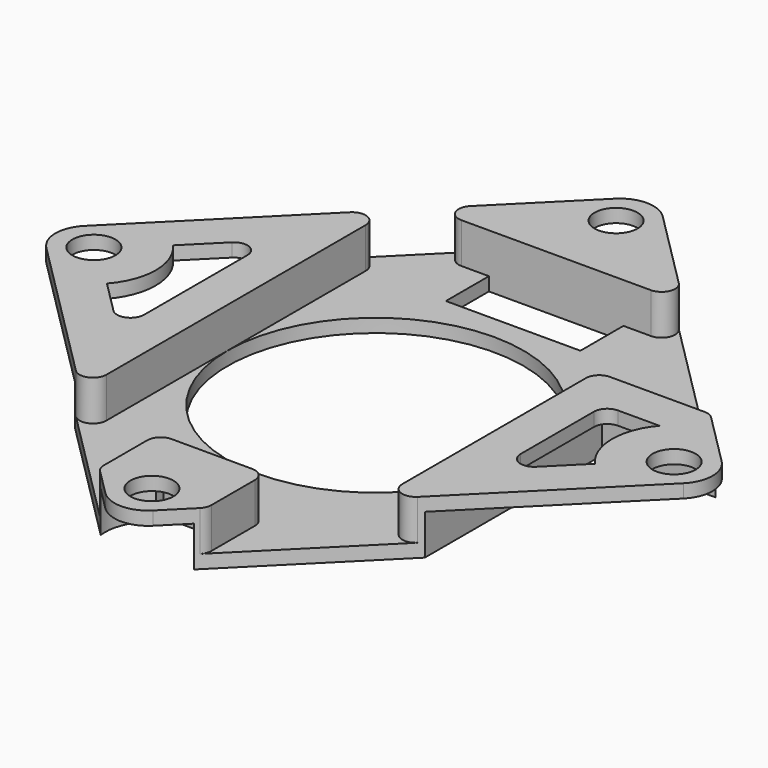
from build123d import *

# Parameters (mm, degrees)
F0_R         = 1.6
F1_DEPTH     = 1
F2_ANGLE     = 45
F3_DEPTH     = 4
F5_DEPTH     = 3
F20_DEPTH    = 3
F7_R         = 11
F8_DEPTH     = 25
F9_DEPTH     = 3
F10_W        = 10
F10_H        = 4
F11_DEPTH    = 25
F13_DEPTH    = 25
F14_DEPTH    = 1
F15_DEPTH    = 2
F16_DEPTH    = 1
F17_DEPTH    = 2
F18_T1_DEPTH = 5.5
F18_T3_DEPTH = 9.0355339059
F18_T5_DEPTH = 4.0355339059


# Not quite as in the source:
# - a fillet or chamfer that OpenCascade refuses, or shapes differently, is made with other operations: its cross-section is extruded or revolved along the edge and cut away or added


with BuildPart() as f1:
    # F0 (on Top) → F1 (new body)
    with BuildSketch(Plane.XY):
        with BuildLine():
            Line((-14.7650561035, -22.9090262799), (16.2349438965, -22.9090262799))
            ThreePointArc((16.2349438965, -22.9090262799), (18.0027108495, -22.1767932329), (18.7349438965, -20.4090262799))
            Line((18.7349438965, -20.4090262799), (18.7349438965, 10.5909737201))
            ThreePointArc((18.7349438965, 10.5909737201), (18.0027108495, 12.3587406731), (16.2349438965, 13.0909737201))
            Line((16.2349438965, 13.0909737201), (-14.7650561035, 13.0909737201))
            ThreePointArc((-14.7650561035, 13.0909737201), (-16.5328230564, 12.3587406731), (-17.2650561035, 10.5909737201))
            Line((-17.2650561035, 10.5909737201), (-17.2650561035, -20.4090262799))
            ThreePointArc((-17.2650561035, -20.4090262799), (-16.5328230564, -22.1767932329), (-14.7650561035, -22.9090262799))
        make_face()
        with Locations((-14.5150561035, -20.1590262799)):
            Circle(F0_R, mode=Mode.SUBTRACT)
        with Locations((15.9849438965, -20.1590262799)):
            Circle(F0_R, mode=Mode.SUBTRACT)
        with Locations((-14.5150561035, 10.3409737201)):
            Circle(F0_R, mode=Mode.SUBTRACT)
        with Locations((15.9849438965, 10.3409737201)):
            Circle(F0_R, mode=Mode.SUBTRACT)
    extrude(amount=F1_DEPTH)


with BuildPart() as f1_1:
    # F2: moved
    add(f1.part.rotate(Axis((16.2349438965, -22.9090262799, 0.5), (0, 0, -1)), F2_ANGLE))

    # F19 (on face) → F3 (join)
    with BuildSketch(Plane.XY.offset(1)):
        Polygon((10.5468667268, -17.2209491102), (25.4585549722, -17.2209491102), (31.0027108495, -11.6767932329), (31.0027108495, 13.2348950126), (25.4585549722, 18.7790508898), (10.5468667268, 18.7790508898), (5.0027108495, 13.2348950126), (5.0027108495, -11.6767932329), align=None)
    extrude(amount=-F3_DEPTH)

    # F4 (on face) → F5 (cut)
    with BuildSketch(Plane.XY.offset(1)):
        Polygon((8.5468667268, -15.2209491102), (27.4585549722, -15.2209491102), (29.0027108495, -13.6767932329), (29.0027108495, 15.2348950126), (27.4585549722, 16.7790508898), (8.5468667268, 16.7790508898), (7.0027108495, 15.2348950126), (7.0027108495, -13.6767932329), align=None)
    extrude(amount=-F5_DEPTH, mode=Mode.SUBTRACT)

    # F6 (on face) → F20 (cut, through all)
    with BuildSketch(Plane.XY.offset(1)):
        Polygon((14.0027108495, -20.6767932329), (14.0027108495, -15.2209491102), (8.5468667268, -15.2209491102), align=None)
        Polygon((27.4585549722, -15.2209491102), (22.0027108495, -15.2209491102), (22.0027108495, -20.6767932329), align=None)
    extrude(amount=-F20_DEPTH, mode=Mode.SUBTRACT)

    # F7 (on face) → F8 (cut)
    with BuildSketch(Plane(origin=(0, 0, -3), x_dir=(1, 0, 0), z_dir=(0, 0, -1))):
        with Locations((18.0027108495, 0)):
            Circle(F7_R)
    extrude(amount=-F8_DEPTH, mode=Mode.SUBTRACT)

    # F21 (on face) → F9 (cut, through all)
    with BuildSketch(Plane.XY.offset(1)):
        Polygon((29.0027108495, 15.2348950126), (29.0027108495, 6.7790508898), (37.4585549722, 6.7790508898), align=None)
    extrude(amount=-F9_DEPTH, mode=Mode.SUBTRACT)

    # F10 (on face) → F11 (cut)
    with BuildSketch(Plane.XY.offset(-2)):
        with Locations((18.0027108495, 14.7790508898)):
            Rectangle(F10_W, F10_H)
    extrude(amount=-F11_DEPTH, mode=Mode.SUBTRACT)

    # F12 (on face) + F22 (on face) → F13 (cut)
    with BuildSketch(Plane.XY.offset(1)):
        with BuildLine():
            ThreePointArc((36.1448070539, -2.2920563414), (34.9697110872, 0.7317293655), (36.0823485209, 3.7790508898))
            Line((36.0823485209, 3.7790508898), (33.0027108495, 3.7790508898))
            ThreePointArc((33.0027108495, 3.7790508898), (32.2956040683, 3.486157671), (32.0027108495, 2.7790508898))
            Line((32.0027108495, 2.7790508898), (32.0027108495, -4.0199389834))
            ThreePointArc((32.0027108495, -4.0199389834), (32.6200274171, -4.9438185159), (33.7098176307, -4.7270457646))
            Line((33.7098176307, -4.7270457646), (36.1448070539, -2.2920563414))
        make_face()
    with BuildSketch(Plane.XY.offset(1)):
        with BuildLine():
            ThreePointArc((-0.1393853549, 3.8501581211), (1.0359540233, 0.7790508898), (-0.1393853549, -2.2920563414))
            Line((-0.1393853549, -2.2920563414), (2.2956040683, -4.7270457646))
            ThreePointArc((2.2956040683, -4.7270457646), (3.3853942819, -4.9438185159), (4.0027108495, -4.0199389834))
            Line((4.0027108495, -4.0199389834), (4.0027108495, 5.5780407631))
            ThreePointArc((4.0027108495, 5.5780407631), (3.3853942819, 6.5019202956), (2.2956040683, 6.2851475443))
            Line((2.2956040683, 6.2851475443), (-0.1393853549, 3.8501581211))
        make_face()
    extrude(amount=-F13_DEPTH, mode=Mode.SUBTRACT)

    # F23 (on face) → F14 (join, through all)
    with BuildSketch(Plane(origin=(0, 0, -3), x_dir=(1, 0, 0), z_dir=(0, 0, -1))):
        with BuildLine():
            Line((14.527236112, 21.2013184954), (10.5468667268, 17.2209491102))
            Line((10.5468667268, 17.2209491102), (16.0027108495, 17.2209491102))
            Line((16.0027108495, 17.2209491102), (16.0027108495, 17.9154246131))
            ThreePointArc((16.0027108495, 17.9154246131), (14.809831185, 19.3539976507), (14.527236112, 21.2013184954))
        make_face()
        with BuildLine():
            Line((20.0027108495, 17.9154246131), (20.0027108495, 17.2209491102))
            Line((20.0027108495, 17.2209491102), (25.4585549722, 17.2209491102))
            Line((25.4585549722, 17.2209491102), (21.478185587, 21.2013184954))
            ThreePointArc((21.478185587, 21.2013184954), (21.195590514, 19.3539976507), (20.0027108495, 17.9154246131))
        make_face()
    extrude(amount=-F14_DEPTH)

    # F24 (on face) → F15 (join, through all)
    with BuildSketch(Plane.XY.offset(-2)):
        with BuildLine():
            Line((22.0027108495, -20.6767932329), (22.0027108495, -17.2209491102))
            Line((22.0027108495, -17.2209491102), (20.0027108495, -17.2209491102))
            Line((20.0027108495, -17.2209491102), (20.0027108495, -17.9154246131))
            ThreePointArc((20.0027108495, -17.9154246131), (21.195590514, -19.3539976507), (21.478185587, -21.2013184954))
            Line((21.478185587, -21.2013184954), (22.0027108495, -20.6767932329))
        make_face()
        with BuildLine():
            Line((16.0027108495, -17.2209491102), (14.0027108495, -17.2209491102))
            Line((14.0027108495, -17.2209491102), (14.0027108495, -20.6767932329))
            Line((14.0027108495, -20.6767932329), (14.527236112, -21.2013184954))
            ThreePointArc((14.527236112, -21.2013184954), (14.809831185, -19.3539976507), (16.0027108495, -17.9154246131))
            Line((16.0027108495, -17.9154246131), (16.0027108495, -17.2209491102))
        make_face()
    extrude(amount=F15_DEPTH)

    # F25 (on face) → F16 (join, through all)
    with BuildSketch(Plane(origin=(0, 0, -3), x_dir=(1, 0, 0), z_dir=(0, 0, -1))):
        Polygon((31.0027108495, -4.7790508898), (31.0027108495, -13.2348950126), (39.4585549722, -4.7790508898), align=None)
    extrude(amount=-F16_DEPTH)

    # F26 (on face) → F17 (join, through all)
    with BuildSketch(Plane.XY.offset(-2)):
        Polygon((37.4585549722, 6.7790508898), (31.0027108495, 6.7790508898), (31.0027108495, 4.7790508898), (39.4585549722, 4.7790508898), align=None)
    extrude(amount=F17_DEPTH)

    # F18: fillet of radius 1 on 11 edges, made by hand

    # F18_s2 → F18_t1 (cut)
    with BuildSketch(Plane.XY.offset(-2)):
        with BuildLine():
            ThreePointArc((22.0027108495, -16.2209491102), (21.7098176307, -15.513842329), (21.0027108495, -15.2209491102))
            Line((21.0027108495, -15.2209491102), (22.0027108495, -15.2209491102))
            Line((22.0027108495, -15.2209491102), (22.0027108495, -16.2209491102))
        make_face()
        with BuildLine():
            ThreePointArc((15.0027108495, -15.2209491102), (14.2956040683, -15.513842329), (14.0027108495, -16.2209491102))
            Line((14.0027108495, -16.2209491102), (14.0027108495, -15.2209491102))
            Line((14.0027108495, -15.2209491102), (15.0027108495, -15.2209491102))
        make_face()
        with BuildLine():
            ThreePointArc((30.0027108495, 6.7790508898), (29.2956040683, 6.486157671), (29.0027108495, 5.7790508898))
            Line((29.0027108495, 5.7790508898), (29.0027108495, 6.7790508898))
            Line((29.0027108495, 6.7790508898), (30.0027108495, 6.7790508898))
        make_face()
    extrude(amount=F18_T1_DEPTH, mode=Mode.SUBTRACT)

    # F18_s4 → F18_t3 (cut)
    with BuildSketch(Plane.XY.offset(-2)):
        with BuildLine():
            ThreePointArc((5.2956040683, -11.9696864517), (6.3853942819, -12.186459203), (7.0027108495, -11.2625796705))
            Line((7.0027108495, -11.2625796705), (7.0027108495, -13.6767932329))
            Line((7.0027108495, -13.6767932329), (5.2956040683, -11.9696864517))
        make_face()
        with BuildLine():
            ThreePointArc((5.2956040683, 13.5277882314), (6.3853942819, 13.7445609827), (7.0027108495, 12.8206814502))
            Line((7.0027108495, 12.8206814502), (7.0027108495, 15.2348950126))
            Line((7.0027108495, 15.2348950126), (5.2956040683, 13.5277882314))
        make_face()
        with BuildLine():
            ThreePointArc((29.0027108495, -11.2625796705), (29.6200274171, -12.186459203), (30.7098176307, -11.9696864517))
            Line((30.7098176307, -11.9696864517), (29.0027108495, -13.6767932329))
            Line((29.0027108495, -13.6767932329), (29.0027108495, -11.2625796705))
        make_face()
        with BuildLine():
            ThreePointArc((10.253973508, 18.486157671), (10.0372007566, 17.3963674575), (10.9610802892, 16.7790508898))
            Line((10.9610802892, 16.7790508898), (8.5468667268, 16.7790508898))
            Line((8.5468667268, 16.7790508898), (10.253973508, 18.486157671))
        make_face()
        with BuildLine():
            ThreePointArc((25.751448191, 18.486157671), (25.9682209424, 17.3963674575), (25.0443414098, 16.7790508898))
            Line((25.0443414098, 16.7790508898), (27.4585549722, 16.7790508898))
            Line((27.4585549722, 16.7790508898), (25.751448191, 18.486157671))
        make_face()
    extrude(amount=F18_T3_DEPTH, mode=Mode.SUBTRACT)

    # F18_s6 → F18_t5 (cut)
    with BuildSketch(Plane.XY.offset(-2)):
        with BuildLine():
            ThreePointArc((14.2956040683, -20.9696864517), (14.078831317, -20.6452631029), (14.0027108495, -20.2625796705))
            Line((14.0027108495, -20.2625796705), (14.0027108495, -20.6767932329))
            Line((14.0027108495, -20.6767932329), (14.2956040683, -20.9696864517))
        make_face()
        with BuildLine():
            ThreePointArc((21.7098176307, -20.9696864517), (21.926590382, -20.6452631029), (22.0027108495, -20.2625796705))
            Line((22.0027108495, -20.2625796705), (22.0027108495, -20.6767932329))
            Line((22.0027108495, -20.6767932329), (21.7098176307, -20.9696864517))
        make_face()
        with BuildLine():
            ThreePointArc((37.751448191, 6.486157671), (37.4270248422, 6.7029304224), (37.0443414098, 6.7790508898))
            Line((37.0443414098, 6.7790508898), (37.4585549722, 6.7790508898))
            Line((37.4585549722, 6.7790508898), (37.751448191, 6.486157671))
        make_face()
    extrude(amount=F18_T5_DEPTH, mode=Mode.SUBTRACT)


solid = f1_1.part
